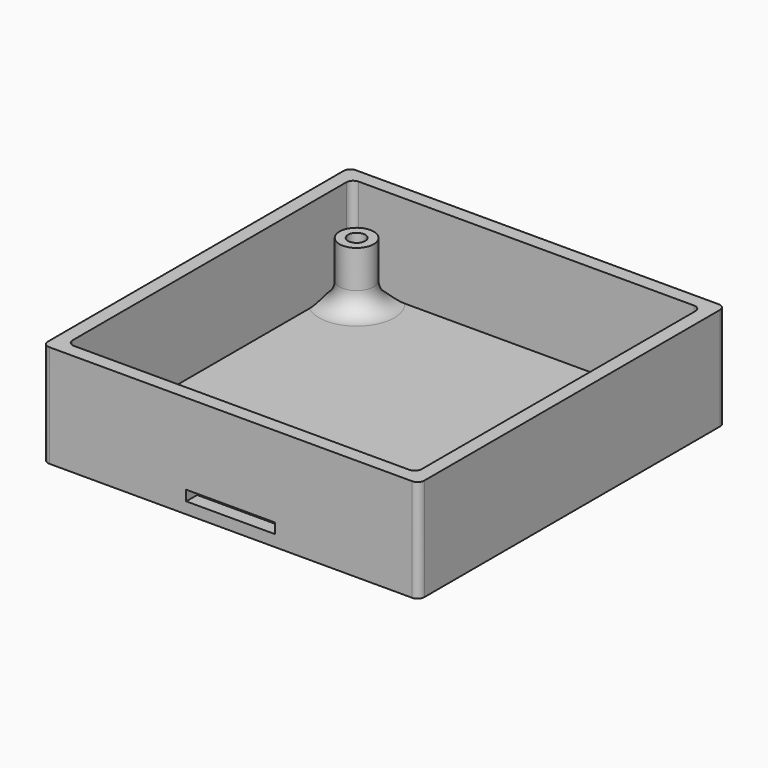
from build123d import *

# Parameters (mm, degrees)
F0_R     = 2.5
F0_R_2   = 1.25
F1_DEPTH = 1.5
F2_DEPTH = 15
F3_DEPTH = 10
F5_W     = 13
F5_H     = 1.5
F6_DEPTH = 5


# Not quite as in the source:
# - a fillet or chamfer that OpenCascade refuses, or shapes differently, is made with other operations: its cross-section is extruded or revolved along the edge and cut away or added


with BuildPart() as f1:
    # F0 (on Top) → F1 (new body)
    with BuildSketch(Plane.XY):
        with BuildLine():
            ThreePointArc((26.5, -28), (27.2071067812, -27.7071067812), (27.5, -27))
            Line((27.5, -27), (27.5, 27))
            ThreePointArc((27.5, 27), (27.2071067812, 27.7071067812), (26.5, 28))
            Line((26.5, 28), (-26.5, 28))
            ThreePointArc((-26.5, 28), (-27.2071067812, 27.7071067812), (-27.5, 27))
            Line((-27.5, 27), (-27.5, -27))
            ThreePointArc((-27.5, -27), (-27.2071067812, -27.7071067812), (-26.5, -28))
            Line((-26.5, -28), (26.5, -28))
        make_face()
        with BuildLine():
            ThreePointArc((25.5, -25), (25.2071067812, -25.7071067812), (24.5, -26))
            Line((24.5, -26), (-24.5, -26))
            ThreePointArc((-24.5, -26), (-25.2071067812, -25.7071067812), (-25.5, -25))
            Line((-25.5, -25), (-25.5, 25))
            ThreePointArc((-25.5, 25), (-25.2071067812, 25.7071067812), (-24.5, 26))
            Line((-24.5, 26), (24.5, 26))
            ThreePointArc((24.5, 26), (25.2071067812, 25.7071067812), (25.5, 25))
            Line((25.5, 25), (25.5, -25))
        make_face(mode=Mode.SUBTRACT)
        with BuildLine():
            Line((-24.5, -26), (24.5, -26))
            ThreePointArc((24.5, -26), (25.2071067812, -25.7071067812), (25.5, -25))
            Line((25.5, -25), (25.5, 25))
            ThreePointArc((25.5, 25), (25.2071067812, 25.7071067812), (24.5, 26))
            Line((24.5, 26), (-24.5, 26))
            ThreePointArc((-24.5, 26), (-25.2071067812, 25.7071067812), (-25.5, 25))
            Line((-25.5, 25), (-25.5, -25))
            ThreePointArc((-25.5, -25), (-25.2071067812, -25.7071067812), (-24.5, -26))
        make_face()
        with Locations((-22, -22.5)):
            Circle(F0_R, mode=Mode.SUBTRACT)
        with Locations((22, -22.5)):
            Circle(F0_R, mode=Mode.SUBTRACT)
        with Locations((-22, 22.5)):
            Circle(F0_R, mode=Mode.SUBTRACT)
        with Locations((22, 22.5)):
            Circle(F0_R, mode=Mode.SUBTRACT)
        with Locations((-22, -22.5)):
            Circle(F0_R)
        with Locations((-22, -22.5)):
            Circle(F0_R_2, mode=Mode.SUBTRACT)
        with Locations((22, -22.5)):
            Circle(F0_R)
        with Locations((22, -22.5)):
            Circle(F0_R_2, mode=Mode.SUBTRACT)
        with Locations((22, 22.5)):
            Circle(F0_R)
        with Locations((22, 22.5)):
            Circle(F0_R_2, mode=Mode.SUBTRACT)
        with Locations((-22, 22.5)):
            Circle(F0_R)
        with Locations((-22, 22.5)):
            Circle(F0_R_2, mode=Mode.SUBTRACT)
        with Locations((-22, -22.5)):
            Circle(F0_R_2)
        with Locations((22, -22.5)):
            Circle(F0_R_2)
        with Locations((22, 22.5)):
            Circle(F0_R_2)
        with Locations((-22, 22.5)):
            Circle(F0_R_2)
    extrude(amount=F1_DEPTH)

    # F0 (on Top) → F2 (join)
    with BuildSketch(Plane.XY):
        with BuildLine():
            ThreePointArc((26.5, -28), (27.2071067812, -27.7071067812), (27.5, -27))
            Line((27.5, -27), (27.5, 27))
            ThreePointArc((27.5, 27), (27.2071067812, 27.7071067812), (26.5, 28))
            Line((26.5, 28), (-26.5, 28))
            ThreePointArc((-26.5, 28), (-27.2071067812, 27.7071067812), (-27.5, 27))
            Line((-27.5, 27), (-27.5, -27))
            ThreePointArc((-27.5, -27), (-27.2071067812, -27.7071067812), (-26.5, -28))
            Line((-26.5, -28), (26.5, -28))
        make_face()
        with BuildLine():
            ThreePointArc((25.5, -25), (25.2071067812, -25.7071067812), (24.5, -26))
            Line((24.5, -26), (-24.5, -26))
            ThreePointArc((-24.5, -26), (-25.2071067812, -25.7071067812), (-25.5, -25))
            Line((-25.5, -25), (-25.5, 25))
            ThreePointArc((-25.5, 25), (-25.2071067812, 25.7071067812), (-24.5, 26))
            Line((-24.5, 26), (24.5, 26))
            ThreePointArc((24.5, 26), (25.2071067812, 25.7071067812), (25.5, 25))
            Line((25.5, 25), (25.5, -25))
        make_face(mode=Mode.SUBTRACT)
    extrude(amount=F2_DEPTH)

    # F0 (on Top) → F3 (join)
    with BuildSketch(Plane.XY):
        with Locations((22, 22.5)):
            Circle(F0_R)
        with Locations((22, 22.5)):
            Circle(F0_R_2, mode=Mode.SUBTRACT)
        with Locations((-22, 22.5)):
            Circle(F0_R)
        with Locations((-22, 22.5)):
            Circle(F0_R_2, mode=Mode.SUBTRACT)
        with Locations((-22, -22.5)):
            Circle(F0_R)
        with Locations((-22, -22.5)):
            Circle(F0_R_2, mode=Mode.SUBTRACT)
        with Locations((22, -22.5)):
            Circle(F0_R)
        with Locations((22, -22.5)):
            Circle(F0_R_2, mode=Mode.SUBTRACT)
    extrude(amount=F3_DEPTH)

    # F4: fillet of radius 3 on 4 edges, made by hand

    # F4_s1 → F4_t2 (revolve)
    with BuildSketch(Plane.XZ.offset(22.5)):
        with BuildLine():
            ThreePointArc((27.5, 1.5), (25.3786796564, 2.3786796564), (24.5, 4.5))
            Line((24.5, 4.5), (24.5, 1.5))
            Line((24.5, 1.5), (27.5, 1.5))
        make_face()
    revolve(axis=Axis((22, -22.5, 1.5), (0, 0, -1)))

    # F4_s3 → F4_t4 (revolve)
    with BuildSketch(Plane.XZ.offset(-22.5)):
        with BuildLine():
            ThreePointArc((-16.5, 1.5), (-18.6213203436, 2.3786796564), (-19.5, 4.5))
            Line((-19.5, 4.5), (-19.5, 1.5))
            Line((-19.5, 1.5), (-16.5, 1.5))
        make_face()
    revolve(axis=Axis((-22, 22.5, 1.5), (0, 0, -1)))

    # F4_s5 → F4_t6 (revolve)
    with BuildSketch(Plane.XZ.offset(22.5)):
        with BuildLine():
            ThreePointArc((-16.5, 1.5), (-18.6213203436, 2.3786796564), (-19.5, 4.5))
            Line((-19.5, 4.5), (-19.5, 1.5))
            Line((-19.5, 1.5), (-16.5, 1.5))
        make_face()
    revolve(axis=Axis((-22, -22.5, 1.5), (0, 0, -1)))

    # F4_s7 → F4_t8 (revolve)
    with BuildSketch(Plane.XZ.offset(-22.5)):
        with BuildLine():
            ThreePointArc((27.5, 1.5), (25.3786796564, 2.3786796564), (24.5, 4.5))
            Line((24.5, 4.5), (24.5, 1.5))
            Line((24.5, 1.5), (27.5, 1.5))
        make_face()
    revolve(axis=Axis((22, 22.5, 1.5), (0, 0, -1)))

    # F5 (on face) → F6 (cut)
    with BuildSketch(Plane.XZ.offset(28)):
        with Locations((0, 2.4238943588)):
            Rectangle(F5_W, F5_H)
    extrude(amount=-F6_DEPTH, mode=Mode.SUBTRACT)


solid = f1.part
